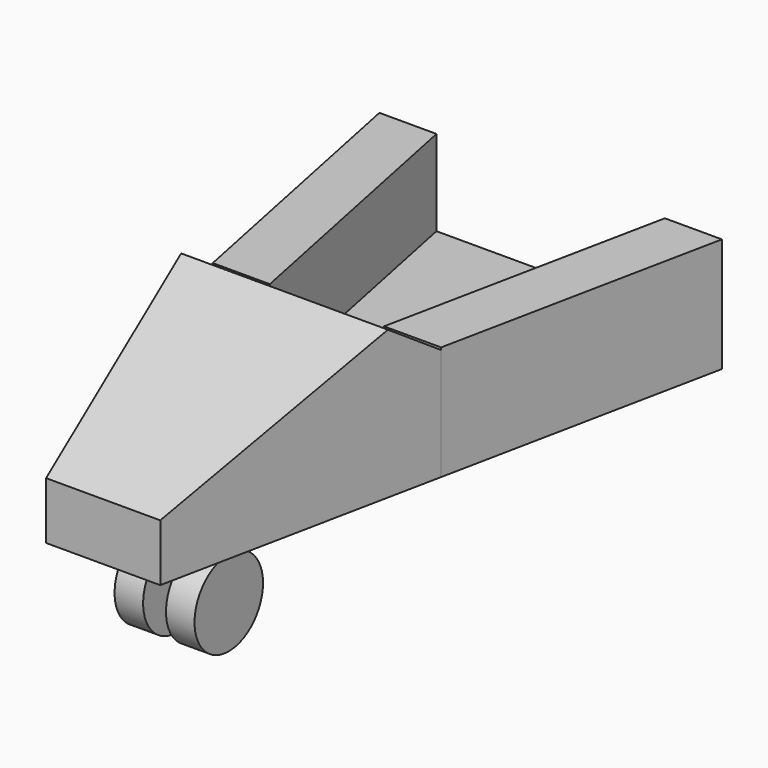
from build123d import *

# Parameters (mm, degrees)
F1_DEPTH    = 25.4
F2_DEPTH    = 38.1
F3_DEPTH    = 6.35
F4_T1_DEPTH = 354.7254321695
F5_SIZE     = 12.7
F6_R        = 9.525
F7_DEPTH    = 3.175


# Not quite as in the source:
# - a fillet or chamfer that OpenCascade refuses, or shapes differently, is made with other operations: its cross-section is extruded or revolved along the edge and cut away or added


with BuildPart() as f1:
    # F0 (on Top) → F1 (new body)
    with BuildSketch(Plane.XY):
        Polygon((-38.432041797, 62.2170394667), (-25.732041797, 0), (-13.032041797, 0), (-25.732041797, 62.2170394667), align=None)
    extrude(amount=F1_DEPTH)


with BuildPart() as f1b:
    # F0 (on Top) → F1, piece 2 (new body)
    with BuildSketch(Plane.XY):
        Polygon((12.367958203, 0), (25.067958203, 0), (37.767958203, 62.2170394667), (25.067958203, 62.2170394667), align=None)
    extrude(amount=F1_DEPTH)


with BuildPart() as f2:
    # F0 (on Top) → F2 (new body)
    with BuildSketch(Plane.XY):
        Polygon((-25.732041797, 0), (-13.032041797, -62.2170394667), (12.367958203, -62.2170394667), (25.067958203, 0), (12.367958203, 0), (-13.032041797, 0), align=None)
    extrude(amount=F2_DEPTH)

    # F4: chamfer of 63.5 x 25.4 on 1 edges, made by hand

    # F4_s2 → F4_t1 (cut)
    with BuildSketch(Plane.YZ.offset(-177.6947578818)):
        Polygon((1.2829605333, 38.1), (-62.2170394667, 12.7), (-62.2170394667, 38.1), align=None)
    extrude(amount=F4_T1_DEPTH, mode=Mode.SUBTRACT)

    # F5
    f5_edges = [f2.edges().sort_by_distance(p)[0] for p in [
        (-0.332042, 0, 37.586816),
    ]]
    chamfer(f5_edges, length=F5_SIZE)


with BuildPart() as f3:
    # F0 (on Top) → F3 (new body)
    with BuildSketch(Plane.XY):
        Polygon((-25.732041797, 62.2170394667), (-13.032041797, 0), (12.367958203, 0), (25.067958203, 62.2170394667), align=None)
    extrude(amount=F3_DEPTH)


with BuildPart() as f7:
    # F6 (on Right) → F7 (new body, symmetric)
    with BuildSketch(Plane.YZ):
        with Locations((-45.9599420428, -9.3141412362)):
            Circle(F6_R)
    extrude(amount=F7_DEPTH, both=True)


with BuildPart() as f8_1:
    # F8: copy of F7
    add(f7.part.moved(Location((11.43, 0, 0))))


solid = Compound([f1.part, f1b.part, f2.part, f3.part, f7.part, f8_1.part])
